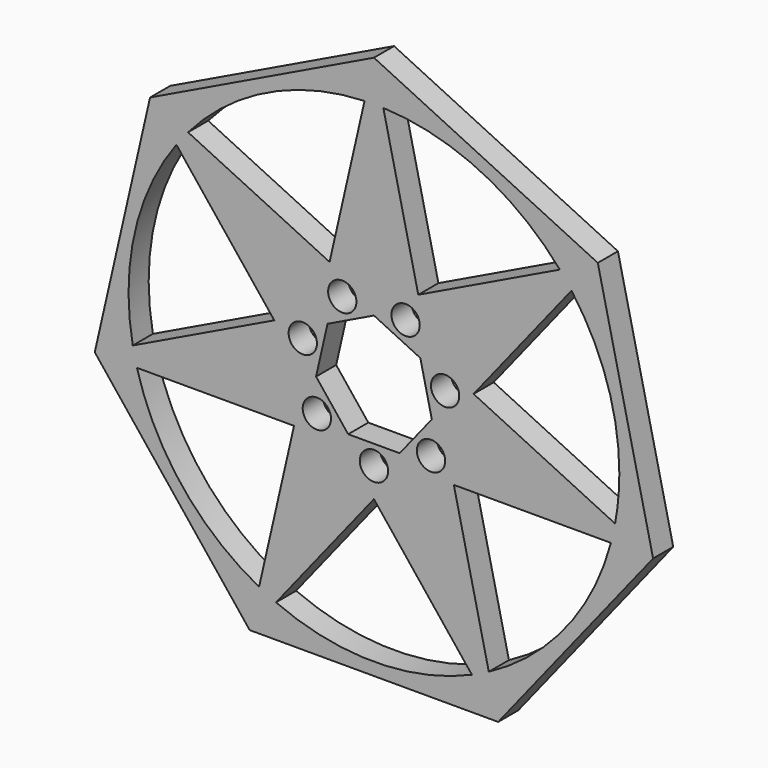
from build123d import *

# Parameters (mm, degrees)
F0_R     = 2.25
F1_DEPTH = 4


# Not quite as in the source:
# - a feature names something its author has since deleted; it is built from what else it names


with BuildPart() as f1:
    # F0 (on Front) → F1 (new body)
    with BuildSketch(Plane.XZ):
        with BuildLine():
            Line((-7.0467516529, 14.6327305836), (-29.539125133, 25.4644867683))
            ThreePointArc((-29.539125133, 25.4644867683), (-30.4914278163, 24.3161022725), (-31.3991126327, 23.1321362152))
            Line((-31.3991126327, 23.1321362152), (-15.8339072365, 3.6139860008))
            Line((-15.8339072365, 3.6139860008), (-8.7871555836, 7.0075227419))
            Line((-8.7871555836, 7.0075227419), (-7.0467516529, 14.6327305836))
        make_face()
        with BuildLine():
            Line((-1.4915941641, 38.9714658032), (-7.0467516529, 14.6327305836))
            Line((-7.0467516529, 14.6327305836), (0, 11.2391938425))
            Line((0, 11.2391938425), (7.0467516529, 14.6327305836))
            Line((7.0467516529, 14.6327305836), (1.4915941641, 38.9714658032))
            ThreePointArc((1.4915941641, 38.9714658032), (0, 39), (-1.4915941641, 38.9714658032))
        make_face()
        Polygon((0, 11.2391938425), (-7.0467516529, 14.6327305836), (-8.7871555836, 7.0075227419), (-15.8339072365, 3.6139860008), (-10.9574037875, -2.5009559107), (-12.6978077182, -10.1261637524), (-4.8765034491, -10.1261637524), (0, -16.241105664), (4.8765034491, -10.1261637524), (12.6978077182, -10.1261637524), (10.9574037875, -2.5009559107), (15.8339072365, 3.6139860008), (8.7871555836, 7.0075227419), (7.0467516529, 14.6327305836), align=None)
        with Locations((-9.0692451966, -7.2324817016)):
            Circle(F0_R, mode=Mode.SUBTRACT)
        with Locations((0, -11.6)):
            Circle(F0_R, mode=Mode.SUBTRACT)
        with Locations((9.0692451966, -7.2324817016)):
            Circle(F0_R, mode=Mode.SUBTRACT)
        with Locations((-11.3091637813, 2.5812428339)):
            Circle(F0_R, mode=Mode.SUBTRACT)
        with Locations((-5.0330513738, 10.4512388677)):
            Circle(F0_R, mode=Mode.SUBTRACT)
        Polygon((-9.1977509421, -2.0993266316), (-7.376023565, 5.8821825089), (0, 9.4342882455), (7.376023565, 5.8821825089), (9.1977509421, -2.0993266316), (4.0933842599, -8.5), (-4.0933842599, -8.5), align=None, mode=Mode.SUBTRACT)
        with Locations((11.3091637813, 2.5812428339)):
            Circle(F0_R, mode=Mode.SUBTRACT)
        with Locations((5.0330513738, 10.4512388677)):
            Circle(F0_R, mode=Mode.SUBTRACT)
        with BuildLine():
            Line((29.539125133, 25.4644867683), (7.0467516529, 14.6327305836))
            Line((7.0467516529, 14.6327305836), (8.7871555836, 7.0075227419))
            Line((8.7871555836, 7.0075227419), (15.8339072365, 3.6139860008))
            Line((15.8339072365, 3.6139860008), (31.3991126327, 23.1321362152))
            ThreePointArc((31.3991126327, 23.1321362152), (30.4914278163, 24.3161022725), (29.539125133, 25.4644867683))
        make_face()
        with BuildLine():
            Line((38.3262807167, -7.2177701839), (15.8339072365, 3.6139860008))
            Line((15.8339072365, 3.6139860008), (10.9574037875, -2.5009559107))
            Line((10.9574037875, -2.5009559107), (12.6978077182, -10.1261637524))
            Line((12.6978077182, -10.1261637524), (37.6624588637, -10.1261637524))
            ThreePointArc((37.6624588637, -10.1261637524), (38.0221885751, -8.6783164243), (38.3262807167, -7.2177701839))
        make_face()
        with BuildLine():
            Line((4.8765034491, -10.1261637524), (0, -16.241105664))
            Line((0, -16.241105664), (15.5652053962, -35.7592558784))
            ThreePointArc((15.5652053962, -35.7592558784), (16.9214658256, -35.1377858482), (18.252965207, -34.464898972))
            Line((18.252965207, -34.464898972), (12.6978077182, -10.1261637524))
            Line((12.6978077182, -10.1261637524), (4.8765034491, -10.1261637524))
        make_face()
        with BuildLine():
            Line((-4.8765034491, -10.1261637524), (-12.6978077182, -10.1261637524))
            Line((-12.6978077182, -10.1261637524), (-18.252965207, -34.464898972))
            ThreePointArc((-18.252965207, -34.464898972), (-16.9214658256, -35.1377858482), (-15.5652053962, -35.7592558784))
            Line((-15.5652053962, -35.7592558784), (0, -16.241105664))
            Line((0, -16.241105664), (-4.8765034491, -10.1261637524))
        make_face()
        with BuildLine():
            Line((-10.9574037875, -2.5009559107), (-15.8339072365, 3.6139860008))
            Line((-15.8339072365, 3.6139860008), (-38.3262807167, -7.2177701839))
            ThreePointArc((-38.3262807167, -7.2177701839), (-38.0221885751, -8.6783164243), (-37.6624588637, -10.1261637524))
            Line((-37.6624588637, -10.1261637524), (-12.6978077182, -10.1261637524))
            Line((-12.6978077182, -10.1261637524), (-10.9574037875, -2.5009559107))
        make_face()
        with BuildLine():
            Line((-29.539125133, 25.4644867683), (-35.5784666076, 28.3728803368))
            Line((-35.5784666076, 28.3728803368), (-31.3991126327, 23.1321362152))
            ThreePointArc((-31.3991126327, 23.1321362152), (-30.4914278163, 24.3161022725), (-29.539125133, 25.4644867683))
        make_face()
        with BuildLine():
            Line((1.4915941641, 38.9714658032), (0, 45.5065668312))
            Line((0, 45.5065668312), (-1.4915941641, 38.9714658032))
            ThreePointArc((-1.4915941641, 38.9714658032), (0, 39), (1.4915941641, 38.9714658032))
        make_face()
        with BuildLine():
            Line((-38.3262807167, -7.2177701839), (-44.3656221913, -10.1261637524))
            Line((-44.3656221913, -10.1261637524), (-37.6624588637, -10.1261637524))
            ThreePointArc((-37.6624588637, -10.1261637524), (-38.0221885751, -8.6783164243), (-38.3262807167, -7.2177701839))
        make_face()
        with BuildLine():
            Line((31.3991126327, 23.1321362152), (35.5784666076, 28.3728803368))
            Line((35.5784666076, 28.3728803368), (29.539125133, 25.4644867683))
            ThreePointArc((29.539125133, 25.4644867683), (30.4914278163, 24.3161022725), (31.3991126327, 23.1321362152))
        make_face()
        with BuildLine():
            Line((37.6624588637, -10.1261637524), (44.3656221913, -10.1261637524))
            Line((44.3656221913, -10.1261637524), (38.3262807167, -7.2177701839))
            ThreePointArc((38.3262807167, -7.2177701839), (38.0221885751, -8.6783164243), (37.6624588637, -10.1261637524))
        make_face()
        with BuildLine():
            Line((15.5652053962, -35.7592558784), (19.7445593711, -41))
            Line((19.7445593711, -41), (18.252965207, -34.464898972))
            ThreePointArc((18.252965207, -34.464898972), (16.9214658256, -35.1377858482), (15.5652053962, -35.7592558784))
        make_face()
        with BuildLine():
            Line((-18.252965207, -34.464898972), (-19.7445593711, -41))
            Line((-19.7445593711, -41), (-15.5652053962, -35.7592558784))
            ThreePointArc((-15.5652053962, -35.7592558784), (-16.9214658256, -35.1377858482), (-18.252965207, -34.464898972))
        make_face()
        with BuildLine():
            Line((0, 45.5065668312), (-35.5784666076, 28.3728803368))
            Line((-35.5784666076, 28.3728803368), (-29.539125133, 25.4644867683))
            ThreePointArc((-29.539125133, 25.4644867683), (-16.9214658256, 35.1377858482), (-1.4915941641, 38.9714658032))
            Line((-1.4915941641, 38.9714658032), (0, 45.5065668312))
        make_face()
        with BuildLine():
            Line((-31.3991126327, 23.1321362152), (-35.5784666076, 28.3728803368))
            Line((-35.5784666076, 28.3728803368), (-44.3656221913, -10.1261637524))
            Line((-44.3656221913, -10.1261637524), (-38.3262807167, -7.2177701839))
            ThreePointArc((-38.3262807167, -7.2177701839), (-38.0221885751, 8.6783164243), (-31.3991126327, 23.1321362152))
        make_face()
        with BuildLine():
            Line((35.5784666076, 28.3728803368), (0, 45.5065668312))
            Line((0, 45.5065668312), (1.4915941641, 38.9714658032))
            ThreePointArc((1.4915941641, 38.9714658032), (16.9214658256, 35.1377858482), (29.539125133, 25.4644867683))
            Line((29.539125133, 25.4644867683), (35.5784666076, 28.3728803368))
        make_face()
        with BuildLine():
            Line((44.3656221913, -10.1261637524), (35.5784666076, 28.3728803368))
            Line((35.5784666076, 28.3728803368), (31.3991126327, 23.1321362152))
            ThreePointArc((31.3991126327, 23.1321362152), (37.051082256, 12.1744529102), (39, 0))
            ThreePointArc((39, 0), (38.8312048999, -3.62457253), (38.3262807167, -7.2177701839))
            Line((38.3262807167, -7.2177701839), (44.3656221913, -10.1261637524))
        make_face()
        with BuildLine():
            Line((19.7445593711, -41), (44.3656221913, -10.1261637524))
            Line((44.3656221913, -10.1261637524), (37.6624588637, -10.1261637524))
            ThreePointArc((37.6624588637, -10.1261637524), (30.4914278163, -24.3161022725), (18.252965207, -34.464898972))
            Line((18.252965207, -34.464898972), (19.7445593711, -41))
        make_face()
        with BuildLine():
            Line((-15.5652053962, -35.7592558784), (-19.7445593711, -41))
            Line((-19.7445593711, -41), (19.7445593711, -41))
            Line((19.7445593711, -41), (15.5652053962, -35.7592558784))
            ThreePointArc((15.5652053962, -35.7592558784), (0, -39), (-15.5652053962, -35.7592558784))
        make_face()
        with BuildLine():
            Line((-37.6624588637, -10.1261637524), (-44.3656221913, -10.1261637524))
            Line((-44.3656221913, -10.1261637524), (-19.7445593711, -41))
            Line((-19.7445593711, -41), (-18.252965207, -34.464898972))
            ThreePointArc((-18.252965207, -34.464898972), (-30.4914278163, -24.3161022725), (-37.6624588637, -10.1261637524))
        make_face()
    extrude(amount=F1_DEPTH)


solid = f1.part
